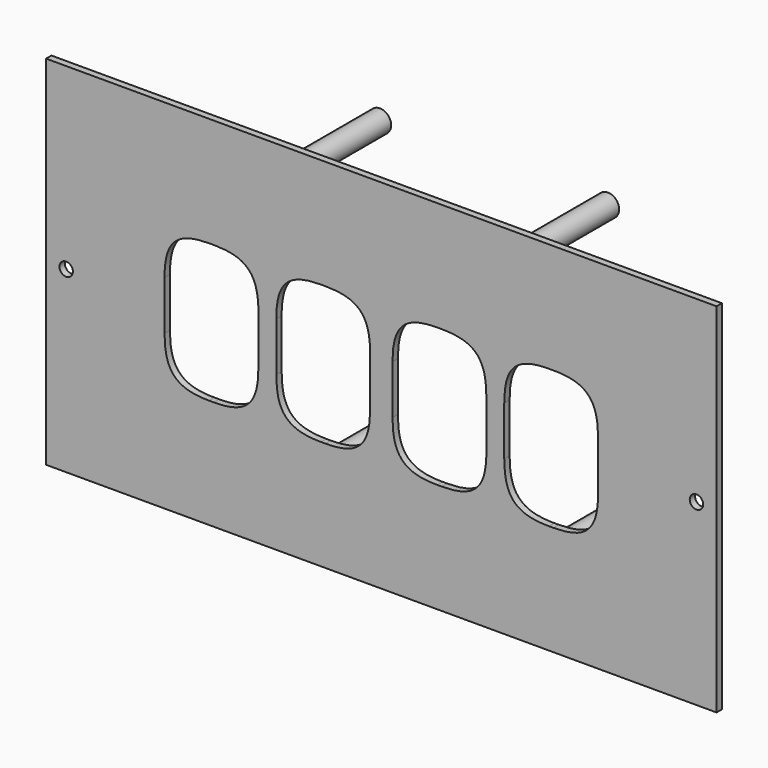
from build123d import *

# Parameters (mm, degrees)
F0_W         = 150
F0_H         = 80
F1_DEPTH     = 1.5
F2_R         = 2.5
F3_DEPTH     = 30
F4_R         = 1.5
F5_R         = 1.5
F6_R         = 1.5
F7_R         = 1.5
F8_DEPTH     = 25
F9_R         = 1.5
F9_W         = 21
F9_H         = 31
F10_DEPTH    = 3
F12_T1_DEPTH = 1.5


# Not quite as in the source:
# - a fillet or chamfer that OpenCascade refuses, or shapes differently, is made with other operations: its cross-section is extruded or revolved along the edge and cut away or added


with BuildPart() as f1:
    # F0 (on Front) → F1 (new body)
    with BuildSketch(Plane.XZ):
        Rectangle(F0_W, F0_H)
    extrude(amount=F1_DEPTH)

    # F2 (on face) → F3 (join)
    with BuildSketch(Plane(origin=(0, 0, 0), x_dir=(-1, 0, 0), z_dir=(0, 1, 0))):
        with Locations((-25.5, 31)):
            Circle(F2_R)
        with Locations((-25.5, -31)):
            Circle(F2_R)
        with Locations((25.5, -31)):
            Circle(F2_R)
        with Locations((25.5, 31)):
            Circle(F2_R)
    extrude(amount=F3_DEPTH)

    # F4 (on face) + F5 (on face) + F6 (on face) + F7 (on face) → F8 (cut)
    with BuildSketch(Plane(origin=(0, 30, 0), x_dir=(-1, 0, 0), z_dir=(0, 1, 0))):
        with Locations((-25.5, 31)):
            Circle(F4_R)
    with BuildSketch(Plane(origin=(0, 30, 0), x_dir=(-1, 0, 0), z_dir=(0, 1, 0))):
        with Locations((25.5, 31)):
            Circle(F5_R)
    with BuildSketch(Plane(origin=(0, 30, 0), x_dir=(-1, 0, 0), z_dir=(0, 1, 0))):
        with Locations((-25.5, -31)):
            Circle(F6_R)
    with BuildSketch(Plane(origin=(0, 30, 0), x_dir=(-1, 0, 0), z_dir=(0, 1, 0))):
        with Locations((25.5, -31)):
            Circle(F7_R)
    extrude(amount=-F8_DEPTH, mode=Mode.SUBTRACT)

    # F9 (on face) → F10 (cut)
    with BuildSketch(Plane.XZ.offset(1.5)):
        with Locations((-70.5, 0)):
            Circle(F9_R)
        with Locations((-38, 0)):
            Rectangle(F9_W, F9_H)
        with Locations((-13, 0)):
            Rectangle(F9_W, F9_H)
    f10 = extrude(amount=-F10_DEPTH, mode=Mode.SUBTRACT)

    # F11: F10 across plane
    add(f10.mirror(Plane.YZ), mode=Mode.SUBTRACT)

    # F12: fillet of radius 10 on 16 edges, made by hand

    # F12_s2 → F12_t1 (join)
    with BuildSketch(Plane.XZ):
        with BuildLine():
            add(Edge.make_bspline(
                [(-38.5, 15.5), (-48.5, 15.5), (-48.5, 5.5)],
                knots=[0, 0, 0, 1, 1, 1], degree=2, weights=[1, 1.2222222222, 1]))
            Line((-48.5, 5.5), (-48.5, 15.5))
            Line((-48.5, 15.5), (-38.5, 15.5))
        make_face()
        with BuildLine():
            add(Edge.make_bspline(
                [(-37.5, 15.5), (-27.5, 15.5), (-27.5, 5.5)],
                knots=[0, 0, 0, 1, 1, 1], degree=2, weights=[1, 1.2222222222, 1]))
            Line((-27.5, 5.5), (-27.5, 15.5))
            Line((-27.5, 15.5), (-37.5, 15.5))
        make_face()
        with BuildLine():
            add(Edge.make_bspline(
                [(-48.5, -5.5), (-48.5, -15.5), (-38.5, -15.5)],
                knots=[0, 0, 0, 1, 1, 1], degree=2, weights=[1, 1.2222222222, 1]))
            Line((-38.5, -15.5), (-48.5, -15.5))
            Line((-48.5, -15.5), (-48.5, -5.5))
        make_face()
        with BuildLine():
            add(Edge.make_bspline(
                [(-27.5, -5.5), (-27.5, -15.5), (-37.5, -15.5)],
                knots=[0, 0, 0, 1, 1, 1], degree=2, weights=[1, 1.2222222222, 1]))
            Line((-37.5, -15.5), (-27.5, -15.5))
            Line((-27.5, -15.5), (-27.5, -5.5))
        make_face()
        with BuildLine():
            add(Edge.make_bspline(
                [(-2.5, -5.5), (-2.5, -15.5), (-12.5, -15.5)],
                knots=[0, 0, 0, 1, 1, 1], degree=2, weights=[1, 1.2222222222, 1]))
            Line((-12.5, -15.5), (-2.5, -15.5))
            Line((-2.5, -15.5), (-2.5, -5.5))
        make_face()
        with BuildLine():
            add(Edge.make_bspline(
                [(-13.5, 15.5), (-23.5, 15.5), (-23.5, 5.5)],
                knots=[0, 0, 0, 1, 1, 1], degree=2, weights=[1, 1.2222222222, 1]))
            Line((-23.5, 5.5), (-23.5, 15.5))
            Line((-23.5, 15.5), (-13.5, 15.5))
        make_face()
        with BuildLine():
            add(Edge.make_bspline(
                [(-23.5, -5.5), (-23.5, -15.5), (-13.5, -15.5)],
                knots=[0, 0, 0, 1, 1, 1], degree=2, weights=[1, 1.2222222222, 1]))
            Line((-13.5, -15.5), (-23.5, -15.5))
            Line((-23.5, -15.5), (-23.5, -5.5))
        make_face()
        with BuildLine():
            add(Edge.make_bspline(
                [(-12.5, 15.5), (-2.5, 15.5), (-2.5, 5.5)],
                knots=[0, 0, 0, 1, 1, 1], degree=2, weights=[1, 1.2222222222, 1]))
            Line((-2.5, 5.5), (-2.5, 15.5))
            Line((-2.5, 15.5), (-12.5, 15.5))
        make_face()
        with BuildLine():
            add(Edge.make_bspline(
                [(23.5, 5.5), (23.5, 15.5), (13.5, 15.5)],
                knots=[0, 0, 0, 1, 1, 1], degree=2, weights=[1, 1.2222222222, 1]))
            Line((13.5, 15.5), (23.5, 15.5))
            Line((23.5, 15.5), (23.5, 5.5))
        make_face()
        with BuildLine():
            add(Edge.make_bspline(
                [(48.5, 5.5), (48.5, 15.5), (38.5, 15.5)],
                knots=[0, 0, 0, 1, 1, 1], degree=2, weights=[1, 1.2222222222, 1]))
            Line((38.5, 15.5), (48.5, 15.5))
            Line((48.5, 15.5), (48.5, 5.5))
        make_face()
        with BuildLine():
            add(Edge.make_bspline(
                [(2.5, -5.5), (2.5, -15.5), (12.5, -15.5)],
                knots=[0, 0, 0, 1, 1, 1], degree=2, weights=[1, 1.2222222222, 1]))
            Line((12.5, -15.5), (2.5, -15.5))
            Line((2.5, -15.5), (2.5, -5.5))
        make_face()
        with BuildLine():
            add(Edge.make_bspline(
                [(27.5, -5.5), (27.5, -15.5), (37.5, -15.5)],
                knots=[0, 0, 0, 1, 1, 1], degree=2, weights=[1, 1.2222222222, 1]))
            Line((37.5, -15.5), (27.5, -15.5))
            Line((27.5, -15.5), (27.5, -5.5))
        make_face()
        with BuildLine():
            add(Edge.make_bspline(
                [(27.5, 5.5), (27.5, 15.5), (37.5, 15.5)],
                knots=[0, 0, 0, 1, 1, 1], degree=2, weights=[1, 1.2222222222, 1]))
            Line((37.5, 15.5), (27.5, 15.5))
            Line((27.5, 15.5), (27.5, 5.5))
        make_face()
        with BuildLine():
            add(Edge.make_bspline(
                [(2.5, 5.5), (2.5, 15.5), (12.5, 15.5)],
                knots=[0, 0, 0, 1, 1, 1], degree=2, weights=[1, 1.2222222222, 1]))
            Line((12.5, 15.5), (2.5, 15.5))
            Line((2.5, 15.5), (2.5, 5.5))
        make_face()
        with BuildLine():
            add(Edge.make_bspline(
                [(38.5, -15.5), (48.5, -15.5), (48.5, -5.5)],
                knots=[0, 0, 0, 1, 1, 1], degree=2, weights=[1, 1.2222222222, 1]))
            Line((48.5, -5.5), (48.5, -15.5))
            Line((48.5, -15.5), (38.5, -15.5))
        make_face()
        with BuildLine():
            add(Edge.make_bspline(
                [(13.5, -15.5), (23.5, -15.5), (23.5, -5.5)],
                knots=[0, 0, 0, 1, 1, 1], degree=2, weights=[1, 1.2222222222, 1]))
            Line((23.5, -5.5), (23.5, -15.5))
            Line((23.5, -15.5), (13.5, -15.5))
        make_face()
    extrude(amount=F12_T1_DEPTH)


solid = f1.part
